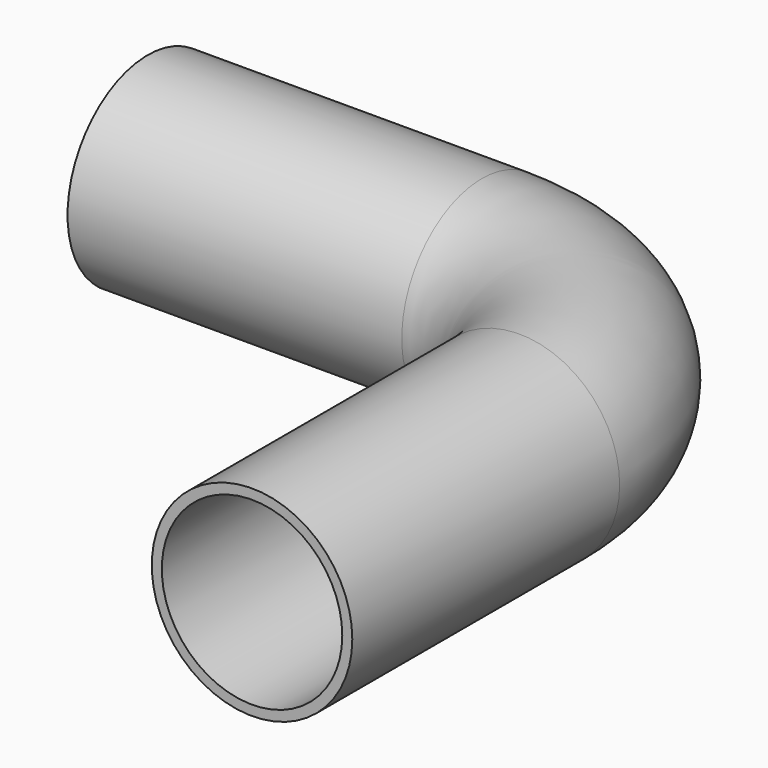
from build123d import *

# Parameters (mm, degrees)
F0_R     = 75
F0_R_2   = 67.5
F5_R     = 7.5
F6_DEPTH = 150


with BuildPart() as f2:
    # F2: sweep along a path in F1
    with BuildLine(Plane.XY) as f2_path:
        Line((0, 0), (0, 250))
        ThreePointArc((0, 250), (-41.0050506339, 348.9949493661), (-140, 390))
        Line((-140, 390), (-390, 390))
    # F0 (on Front) → F2 (sweep)
    with BuildSketch(Plane.XZ):
        Circle(F0_R)
        Circle(F0_R_2, mode=Mode.SUBTRACT)
    sweep(path=f2_path.line)

    # F5 (on face) → F6 (cut)
    with BuildSketch(Plane(origin=(267.132034356, 267.132034356, 0), x_dir=(-0.7071067812, 0.7071067812, 0), z_dir=(0.7071067812, 0.7071067812, 0))):
        with Locations((276.0982438922, 0)):
            Circle(F5_R)
    extrude(amount=-F6_DEPTH, mode=Mode.SUBTRACT)


solid = f2.part
